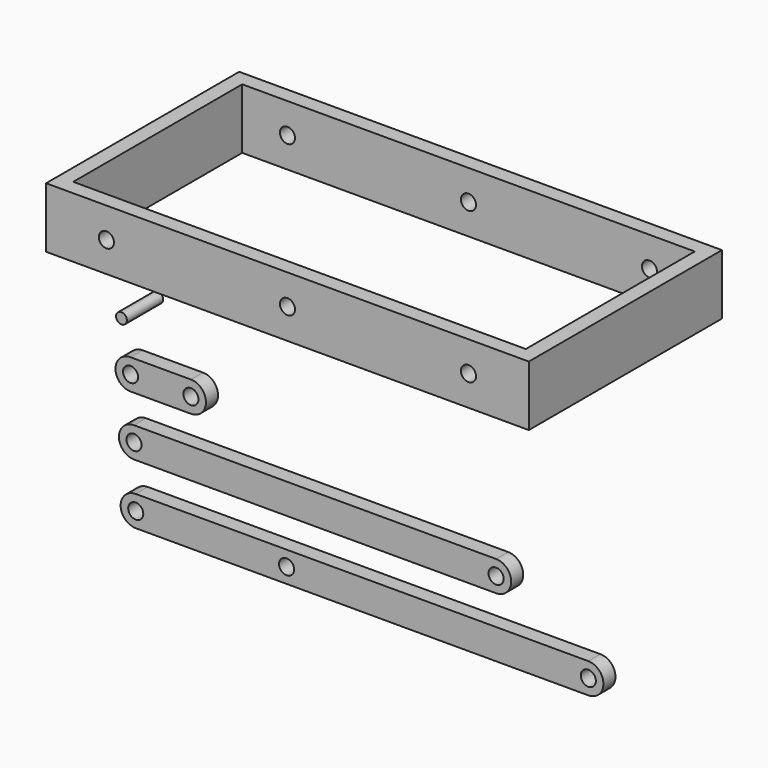
from build123d import *

# Parameters (mm, degrees)
F1_R      = 1.25
F2_DEPTH  = 2.5
F3_R      = 1.25
F4_DEPTH  = 2.5
F5_R      = 1.25
F6_DEPTH  = 2.5
F8_W      = 80
F8_H      = 40
F8_W_2    = 75
F8_H_2    = 35
F9_DEPTH  = 10
F10_R     = 1.25
F11_DEPTH = 40.001
F12_R     = 0.9
F13_DEPTH = 7.5


with BuildPart() as f2:
    # F1 (on Front) → F2 (new body)
    with BuildSketch(Plane.XZ):
        with BuildLine():
            Line((10, 2.5), (0, 2.5))
            ThreePointArc((0, 2.5), (-2.5, 0), (0, -2.5))
            Line((0, -2.5), (10, -2.5))
            ThreePointArc((10, -2.5), (12.5, 0), (10, 2.5))
        make_face()
        Circle(F1_R, mode=Mode.SUBTRACT)
        with Locations((10, 0)):
            Circle(F1_R, mode=Mode.SUBTRACT)
    extrude(amount=F2_DEPTH)


with BuildPart() as f4:
    # F3 (on Front) → F4 (new body)
    with BuildSketch(Plane.XZ):
        with BuildLine():
            Line((60.5706622079, -7.232673876), (0.5706622079, -7.232673876))
            ThreePointArc((0.5706622079, -7.232673876), (-1.9293377921, -9.732673876), (0.5706622079, -12.232673876))
            Line((0.5706622079, -12.232673876), (60.5706622079, -12.232673876))
            ThreePointArc((60.5706622079, -12.232673876), (63.0706622079, -9.732673876), (60.5706622079, -7.232673876))
        make_face()
        with Locations((0.5706622079, -9.732673876)):
            Circle(F3_R, mode=Mode.SUBTRACT)
        with Locations((60.5706622079, -9.732673876)):
            Circle(F3_R, mode=Mode.SUBTRACT)
    extrude(amount=F4_DEPTH)


with BuildPart() as f6:
    # F5 (on Front) → F6 (new body)
    with BuildSketch(Plane.XZ):
        with BuildLine():
            Line((75.8570737601, -17.1626018733), (0.8570737601, -17.1626018733))
            ThreePointArc((0.8570737601, -17.1626018733), (-1.6429262399, -19.6626018733), (0.8570737601, -22.1626018733))
            Line((0.8570737601, -22.1626018733), (75.8570737601, -22.1626018733))
            ThreePointArc((75.8570737601, -22.1626018733), (78.3570737601, -19.6626018733), (75.8570737601, -17.1626018733))
        make_face()
        with Locations((0.8570737601, -19.6626018733)):
            Circle(F5_R, mode=Mode.SUBTRACT)
        with Locations((25.8570737601, -19.6626018733)):
            Circle(F5_R, mode=Mode.SUBTRACT)
        with Locations((75.8570737601, -19.6626018733)):
            Circle(F5_R, mode=Mode.SUBTRACT)
    extrude(amount=F6_DEPTH)


with BuildPart() as f9:
    # F8 (on offset) → F9 (new body)
    with BuildSketch(Plane.XY.offset(25)):
        with Locations((40, 0)):
            Rectangle(F8_W, F8_H)
        with Locations((40, 0)):
            Rectangle(F8_W_2, F8_H_2, mode=Mode.SUBTRACT)
    extrude(amount=F9_DEPTH)

    # F10 (on face) → F11 (cut, through all)
    with BuildSketch(Plane.XZ.offset(20)):
        with Locations((10, 30)):
            Circle(F10_R)
        with Locations((70, 30)):
            Circle(F10_R)
        with Locations((40, 30)):
            Circle(F10_R)
    extrude(amount=-F11_DEPTH, mode=Mode.SUBTRACT)


with BuildPart() as f13:
    # F12 (on Front) → F13 (new body)
    with BuildSketch(Plane.XZ):
        with Locations((2.488047583, 11.0218990594)):
            Circle(F12_R)
    extrude(amount=F13_DEPTH)


solid = Compound([f2.part, f4.part, f6.part, f9.part, f13.part])
